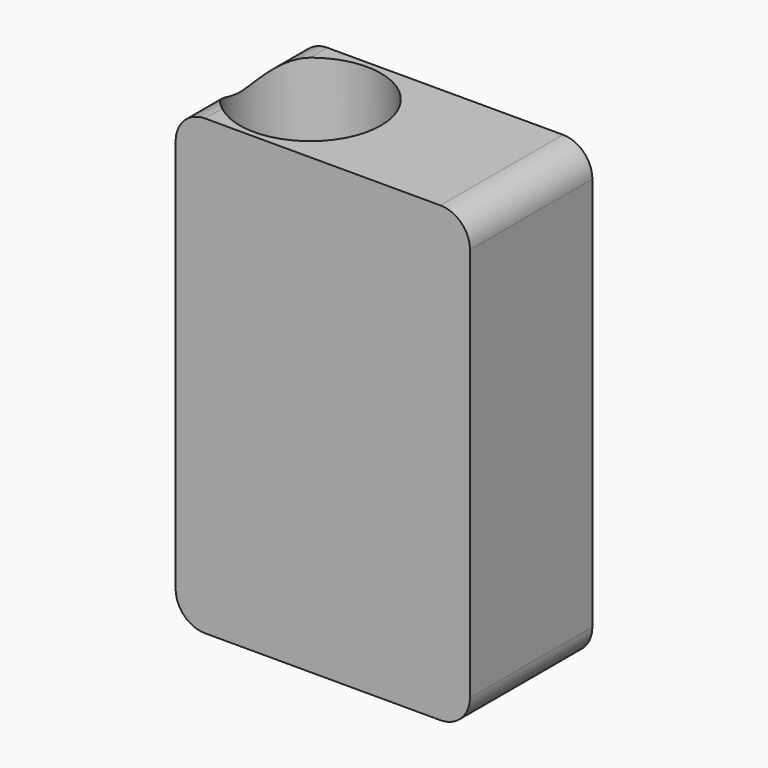
from build123d import *

# Parameters (mm, degrees)
F0_W     = 50
F0_H     = 26
F1_DEPTH = 77
F2_R     = 5
F4_DEPTH = 25


with BuildPart() as f1:
    # F0 (on Top) → F1 (new body)
    with BuildSketch(Plane.XY):
        Rectangle(F0_W, F0_H)
    extrude(amount=F1_DEPTH)

    # F2
    f2_edges = [f1.edges().sort_by_distance(p)[0] for p in [
        (-25, 0, 0),
        (25, 0, 0),
        (-25, 0, 77),
        (25, 0, 77),
    ]]
    fillet(f2_edges, radius=F2_R)

    # F3 (on face) → F4 (cut)
    with BuildSketch(Plane.XY.offset(77)):
        with BuildLine():
            ThreePointArc((-20, -9.3674969976), (-7.3038475773, -10.8166538264), (-0.5, 0))
            ThreePointArc((-0.5, 0), (-7.3038475773, 10.8166538264), (-20, 9.3674969976))
            Line((-20, 9.3674969976), (-20, -9.3674969976))
        make_face()
        with BuildLine():
            Line((-20, -9.3674969976), (-20, 9.3674969976))
            ThreePointArc((-20, 9.3674969976), (-24.5, 0), (-20, -9.3674969976))
        make_face()
    extrude(amount=-F4_DEPTH, mode=Mode.SUBTRACT)


solid = f1.part
